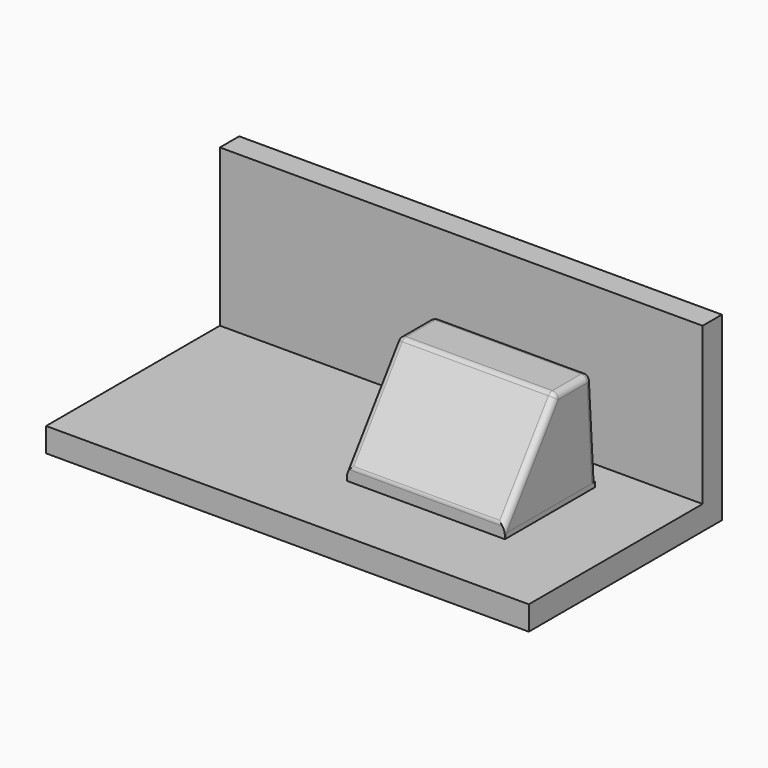
from build123d import *

# Parameters (mm, degrees)
F1_DEPTH     = 200
F2_W         = 131
F2_H         = 92
F3_DEPTH     = 4
F5_DEPTH     = 131
F6_T1_DEPTH  = 100.6767614544
F6_T3_DEPTH  = 139.007901378
F6_T5_DEPTH  = 121
F6_T7_DEPTH  = 88.2624487626
F6_T9_DEPTH  = 29.9131719037
F6_T14_DEPTH = 5
F6_T20_DEPTH = 5
F6_T26_DEPTH = 5
F6_T32_DEPTH = 5


# Not quite as in the source:
# - a fillet or chamfer that OpenCascade refuses, or shapes differently, is made with other operations: its cross-section is extruded or revolved along the edge and cut away or added
# - two fillets or chamfers of one size are made in one step


with BuildPart() as f1:
    # F0 (on Right) → F1 (new body, symmetric)
    with BuildSketch(Plane.YZ):
        Polygon((0, 0), (-180, 0), (-180, -20), (20, -20), (20, 130), (0, 130), align=None)
    extrude(amount=F1_DEPTH, both=True)


with BuildPart() as f3:
    # F2 (on face) → F3 (new body)
    with BuildSketch(Plane.XY):
        with Locations((65.5, -71)):
            Rectangle(F2_W, F2_H)
    extrude(amount=F3_DEPTH)


with BuildPart() as f5:
    # F4 (on Right) → F5 (new body, through all)
    with BuildSketch(Plane.YZ):
        Polygon((-117, 3.9981720038), (-25, 4), (-25, 0), (-23.5, 0), (-23.5, 4.0475159867), (-28.5921140468, 84.3416133777), (-65.772183231, 84.3416133777), (-118.5, 10.4804740827), (-118.5, 0), (-116.9999205582, 0), align=None)
    extrude(amount=F5_DEPTH)

    # F6: fillet of radius 5 on 9 edges, made by hand

    # F6_s2 → F6_t1 (cut)
    with BuildSketch(Plane(origin=(0, 16.184877417, 22.6717804496), x_dir=(1, 0, 0), z_dir=(0, -0.581018257, -0.8138905239))):
        with BuildLine():
            ThreePointArc((5, 102.5353738726), (1.4644660941, 101.0709077785), (0, 97.5353738726))
            Line((0, 97.5353738726), (0, 102.5353738726))
            Line((0, 102.5353738726), (5, 102.5353738726))
        make_face()
        with BuildLine():
            ThreePointArc((126, 102.5353738726), (129.5355339059, 101.0709077785), (131, 97.5353738726))
            Line((131, 97.5353738726), (131, 102.5353738726))
            Line((131, 102.5353738726), (126, 102.5353738726))
        make_face()
    extrude(amount=F6_T1_DEPTH, mode=Mode.SUBTRACT)

    # F6_s4 → F6_t3 (cut)
    with BuildSketch(Plane.YZ.offset(-4.003950689)):
        with BuildLine():
            ThreePointArc((-117.5694526197, 11.7839850923), (-118.2616836885, 10.4041375419), (-118.5, 8.8788938071))
            Line((-118.5, 8.8788938071), (-118.5, 10.4804740827))
            Line((-118.5, 10.4804740827), (-117.5694526197, 11.7839850923))
        make_face()
    extrude(amount=F6_T3_DEPTH, mode=Mode.SUBTRACT)

    # F6_s6 → F6_t5 (cut)
    with BuildSketch(Plane.YZ.offset(5)):
        with BuildLine():
            ThreePointArc((-63.1982391278, 84.3416133777), (-65.4867477659, 83.7871423916), (-67.2676917475, 82.246704663))
            Line((-67.2676917475, 82.246704663), (-65.772183231, 84.3416133777))
            Line((-65.772183231, 84.3416133777), (-63.1982391278, 84.3416133777))
        make_face()
        with BuildLine():
            ThreePointArc((-28.2950916938, 79.6580690739), (-29.8632459605, 82.9873148521), (-33.2850672241, 84.3416133777))
            Line((-33.2850672241, 84.3416133777), (-28.5921140468, 84.3416133777))
            Line((-28.5921140468, 84.3416133777), (-28.2950916938, 79.6580690739))
        make_face()
    extrude(amount=F6_T5_DEPTH, mode=Mode.SUBTRACT)

    # F6_s8 → F6_t7 (cut)
    with BuildSketch(Plane(origin=(0, 0.4413453849, -6.9592764405), x_dir=(1, 0, 0), z_dir=(0, -0.0632911392, 0.997995106))):
        with BuildLine():
            ThreePointArc((5, -23.1967130942), (1.4644660941, -24.6611791883), (0, -28.1967130942))
            Line((0, -28.1967130942), (0, -23.1967130942))
            Line((0, -23.1967130942), (5, -23.1967130942))
        make_face()
        with BuildLine():
            ThreePointArc((126, -23.1967130942), (129.5355339059, -24.6611791883), (131, -28.1967130942))
            Line((131, -28.1967130942), (131, -23.1967130942))
            Line((131, -23.1967130942), (126, -23.1967130942))
        make_face()
    extrude(amount=F6_T7_DEPTH, mode=Mode.SUBTRACT)

    # F6_s10 → F6_t9 (cut)
    with BuildSketch(Plane.XZ.offset(33.2850672241)):
        with BuildLine():
            ThreePointArc((5, 84.3416133777), (1.4644660941, 82.8771472836), (0, 79.3416133777))
            Line((0, 79.3416133777), (0, 84.3416133777))
            Line((0, 84.3416133777), (5, 84.3416133777))
        make_face()
        with BuildLine():
            ThreePointArc((126, 84.3416133777), (129.5355339059, 82.8771472836), (131, 79.3416133777))
            Line((131, 79.3416133777), (131, 84.3416133777))
            Line((131, 84.3416133777), (126, 84.3416133777))
        make_face()
    extrude(amount=F6_T9_DEPTH, mode=Mode.SUBTRACT)


with BuildPart() as f6_tool12:
    # F6_s13 → F6_t14 (new body)
    with BuildSketch(Plane.YZ.offset(5)):
        Polygon((-63.1982391278, 79.3416133777), (-63.1982391278, 84.3416133777), (-65.772183231, 84.3416133777), (-67.2676917475, 82.246704663), align=None)
    extrude(amount=-F6_T14_DEPTH)

    # F6_s15 → F6_t16 (revolve, cut)
    with BuildSketch(Plane(origin=(5, -63.1982391278, 79.3416133777), x_dir=(0, 0.4577017276, -0.8891058028), z_dir=(0, 0.8891058028, 0.4577017276))):
        with BuildLine():
            ThreePointArc((0, -5), (5, 0), (0, 5))
            Line((0, 5), (0, -5))
        make_face()
    revolve(axis=Axis((5, -63.1982391278, 79.3416133777), (-1, 0, 0)), mode=Mode.SUBTRACT)


with BuildPart() as f5_1:
    add(f5.part)

    # F6_t11: cut F6_tool12
    add(f6_tool12.part, mode=Mode.SUBTRACT)


with BuildPart() as f6_tool18:
    # F6_s19 → F6_t20 (new body)
    with BuildSketch(Plane.YZ.offset(126)):
        Polygon((-63.1982391278, 79.3416133777), (-63.1982391278, 84.3416133777), (-65.772183231, 84.3416133777), (-67.2676917475, 82.246704663), align=None)
    extrude(amount=F6_T20_DEPTH)

    # F6_s21 → F6_t22 (revolve, cut)
    with BuildSketch(Plane(origin=(126, -63.1982391278, 79.3416133777), x_dir=(0, 0.4577017276, -0.8891058028), z_dir=(0, -0.8891058028, -0.4577017276))):
        with BuildLine():
            ThreePointArc((0, -5), (5, 0), (0, 5))
            Line((0, 5), (0, -5))
        make_face()
    revolve(axis=Axis((126, -63.1982391278, 79.3416133777), (1, 0, 0)), mode=Mode.SUBTRACT)


with BuildPart() as f5_2:
    add(f5_1.part)

    # F6_t17: cut F6_tool18
    add(f6_tool18.part, mode=Mode.SUBTRACT)


with BuildPart() as f6_tool24:
    # F6_s25 → F6_t26 (new body)
    with BuildSketch(Plane.YZ.offset(5)):
        Polygon((-33.2850672241, 79.3416133777), (-28.2950916938, 79.6580690739), (-28.5921140468, 84.3416133777), (-33.2850672241, 84.3416133777), align=None)
    extrude(amount=-F6_T26_DEPTH)

    # F6_s27 → F6_t28 (revolve, cut)
    with BuildSketch(Plane(origin=(5, -33.2850672241, 79.3416133777), x_dir=(0, -0.6843642527, -0.7291402949), z_dir=(0, 0.7291402949, -0.6843642527))):
        with BuildLine():
            ThreePointArc((0, -5), (5, 0), (0, 5))
            Line((0, 5), (0, -5))
        make_face()
    revolve(axis=Axis((5, -33.2850672241, 79.3416133777), (-1, 0, 0)), mode=Mode.SUBTRACT)


with BuildPart() as f5_3:
    add(f5_2.part)

    # F6_t23: cut F6_tool24
    add(f6_tool24.part, mode=Mode.SUBTRACT)


with BuildPart() as f6_tool30:
    # F6_s31 → F6_t32 (new body)
    with BuildSketch(Plane.YZ.offset(126)):
        Polygon((-33.2850672241, 79.3416133777), (-28.2950916938, 79.6580690739), (-28.5921140468, 84.3416133777), (-33.2850672241, 84.3416133777), align=None)
    extrude(amount=F6_T32_DEPTH)

    # F6_s33 → F6_t34 (revolve, cut)
    with BuildSketch(Plane(origin=(126, -33.2850672241, 79.3416133777), x_dir=(0, -0.6843642527, -0.7291402949), z_dir=(0, -0.7291402949, 0.6843642527))):
        with BuildLine():
            ThreePointArc((0, -5), (5, 0), (0, 5))
            Line((0, 5), (0, -5))
        make_face()
    revolve(axis=Axis((126, -33.2850672241, 79.3416133777), (1, 0, 0)), mode=Mode.SUBTRACT)


with BuildPart() as f5_4:
    add(f5_3.part)

    # F6_t29: cut F6_tool30
    add(f6_tool30.part, mode=Mode.SUBTRACT)


solid = Compound([f1.part, f3.part, f5_4.part])
